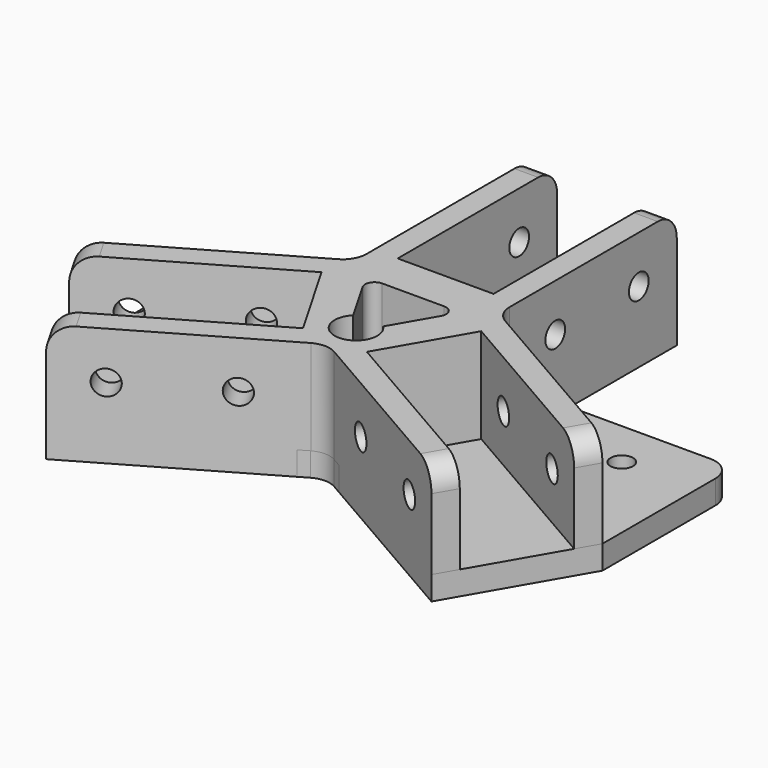
from build123d import *

# Parameters (mm, degrees)
F1_DEPTH    = 20
F2_R        = 2.6
F3_DEPTH    = 50.6016350946
F4_COUNT    = 3
F4_ANGLE    = 240
F6_DEPTH    = 5
F7_T1_DEPTH = 25
F10_DEPTH   = 5
F11_DEPTH   = 25.001
F12_R       = 2
F13_R       = 2.6
F13_R_2     = 2.372590354
F14_DEPTH   = 25.001
F15_R       = 5
F16_R       = 4.5
F17_DEPTH   = 20


# Not quite as in the source:
# - a fillet or chamfer that OpenCascade refuses, or shapes differently, is made with other operations: its cross-section is extruded or revolved along the edge and cut away or added


with BuildPart() as f1:
    # F0 (on Top) → F1 (new body)
    with BuildSketch(Plane.XY):
        Polygon((43.0992290895, -36.5458269543), (6.7261621305, -15.5458269543), (16.8261621305, 1.9478862021), (53.1992290895, -19.0521137979), (55.6992290895, -14.7219867789), (14.8979589003, 8.8346375481), (0, 0), (-0.2020410997, -17.3193296462), (40.5992290895, -40.8759539732), align=None)
    extrude(amount=F1_DEPTH)

    # F2 (on face) → F3 (cut, through all)
    with BuildSketch(Plane(origin=(-7.55, -13.0769835971, 0), x_dir=(0.8660254038, -0.5, 0), z_dir=(-0.5, -0.8660254038, 0))):
        with Locations((45.5979407522, 10)):
            Circle(F2_R)
        with Locations((23.5979407522, 10)):
            Circle(F2_R)
    extrude(amount=-F3_DEPTH, mode=Mode.SUBTRACT)

    # F4: F1 ×3 about axis
    f4_axis = Axis((0, 0, 10), (0, 0, -1))


with BuildPart() as f1_1:
    add(f1.part)
    for i in range(1, F4_COUNT):
        add(f1.part.rotate(f4_axis, i * F4_ANGLE / (F4_COUNT - 1)))

    # F5 (on face) → F6 (join)
    with BuildSketch(Plane(origin=(0, 0, 0), x_dir=(1, 0, 0), z_dir=(0, 0, -1))):
        Polygon((0, 17.4359781295), (-40.5992290895, 40.8759539732), (-55.6992290895, 14.7219867789), (-15.1, -8.7179890648), (-15.1, -55.5979407522), (15.1, -55.5979407522), (15.1, -8.7179890648), (55.6992290895, 14.7219867789), (40.5992290895, 40.8759539732), align=None)
    extrude(amount=F6_DEPTH)

    # F7: fillet of radius 5 on 3 edges, made by hand

    # F7_s2 → F7_t1 (join)
    with BuildSketch(Plane.XY.offset(-5)):
        with BuildLine():
            ThreePointArc((2.5012, -18.8795847426), (0, -18.2093902225), (-2.5012, -18.8795847426))
            Line((-2.5012, -18.8795847426), (-2.75132, -18.4463641946))
            ThreePointArc((-2.75132, -18.4463641946), (-1.50062, -17.7247340932), (-0.25012, -17.0027575815))
            Line((-0.25012, -17.0027575815), (0.25012, -17.0027575815))
            ThreePointArc((0.25012, -17.0027575815), (1.50062, -17.7247340932), (2.75132, -18.4463641946))
            Line((2.75132, -18.4463641946), (2.5012, -18.8795847426))
        make_face()
        with BuildLine():
            ThreePointArc((15.0996, 11.6058951112), (15.7697945201, 9.1046951112), (17.6008, 7.2736896314))
            Line((17.6008, 7.2736896314), (17.35068, 6.8404690834))
            ThreePointArc((17.35068, 6.8404690834), (16.10038, 7.5627920052), (14.84988, 8.2847685168))
            Line((14.84988, 8.2847685168), (14.59976, 8.7179890648))
            ThreePointArc((14.59976, 8.7179890648), (14.59976, 10.161942088), (14.59936, 11.6058951112))
            Line((14.59936, 11.6058951112), (15.0996, 11.6058951112))
        make_face()
        with BuildLine():
            ThreePointArc((-17.6008, 7.2736896314), (-15.7697945201, 9.1046951112), (-15.0996, 11.6058951112))
            Line((-15.0996, 11.6058951112), (-14.59936, 11.6058951112))
            ThreePointArc((-14.59936, 11.6058951112), (-14.59976, 10.161942088), (-14.59976, 8.7179890648))
            Line((-14.59976, 8.7179890648), (-14.84988, 8.2847685168))
            ThreePointArc((-14.84988, 8.2847685168), (-16.10038, 7.5627920052), (-17.35068, 6.8404690834))
            Line((-17.35068, 6.8404690834), (-17.6008, 7.2736896314))
        make_face()
    extrude(amount=F7_T1_DEPTH)

    # F9 (on face) → F10 (join)
    with BuildSketch(Plane(origin=(0, 0, -5), x_dir=(1, 0, 0), z_dir=(0, 0, -1))):
        with BuildLine():
            Line((-55.6992290895, 14.7219867789), (-55.6992290895, -20))
            Line((-55.6992290895, -20), (55.6992290895, -20))
            Line((55.6992290895, -20), (55.6992290895, 14.7219867789))
            Line((55.6992290895, 14.7219867789), (52.6519667355, 20))
            Line((52.6519667355, 20), (4.4410161514, 20))
            Line((4.4410161514, 20), (2.5, 18.8793538025))
            ThreePointArc((2.5, 18.8793538025), (0, 18.2094808214), (-2.5, 18.8793538025))
            Line((-2.5, 18.8793538025), (-4.4410161514, 20))
            Line((-4.4410161514, 20), (-52.6519667355, 20))
            Line((-52.6519667355, 20), (-55.6992290895, 14.7219867789))
        make_face()
    extrude(amount=-F10_DEPTH)

    # F8 (on face) → F11 (cut, through all)
    with BuildSketch(Plane.XY.offset(20)):
        Polygon((10, 5.0614941438), (-10, 5.0614941438), (0, -12.2590139319), align=None)
    extrude(amount=-F11_DEPTH, mode=Mode.SUBTRACT)

    # F12
    f12_edges = [f1_1.edges().sort_by_distance(p)[0] for p in [
        (10, 5.061494, 7.5),
        (-10, 5.061494, 7.5),
        (0, -12.259014, 7.5),
    ]]
    fillet(f12_edges, radius=F12_R)

    # F13 (on face) → F14 (cut, through all)
    with BuildSketch(Plane(origin=(0, 0, -5), x_dir=(1, 0, 0), z_dir=(0, 0, -1))):
        with Locations((-40, -10)):
            Circle(F13_R)
        with Locations((40, -10)):
            Circle(F13_R_2)
        with Locations((0, 10)):
            Circle(F13_R)
    extrude(amount=-F14_DEPTH, mode=Mode.SUBTRACT)

    # F15
    f15_edges = [f1_1.edges().sort_by_distance(p)[0] for p in [
        (-15.1, 20, -2.5),
        (15.1, 20, -2.5),
        (55.699229, 20, -2.5),
        (-55.699229, 20, -2.5),
        (-12.6, 55.597941, 20),
        (12.6, 55.597941, 20),
        (-54.449229, -16.88705, 20),
        (-41.849229, -38.71089, 20),
        (54.449229, -16.88705, 20),
        (41.849229, -38.71089, 20),
    ]]
    fillet(f15_edges, radius=F15_R)

    # F16 (on face) → F17 (cut)
    with BuildSketch(Plane.XY.offset(20)):
        with Locations((0, -10)):
            Circle(F16_R)
    extrude(amount=-F17_DEPTH, mode=Mode.SUBTRACT)


solid = f1_1.part
